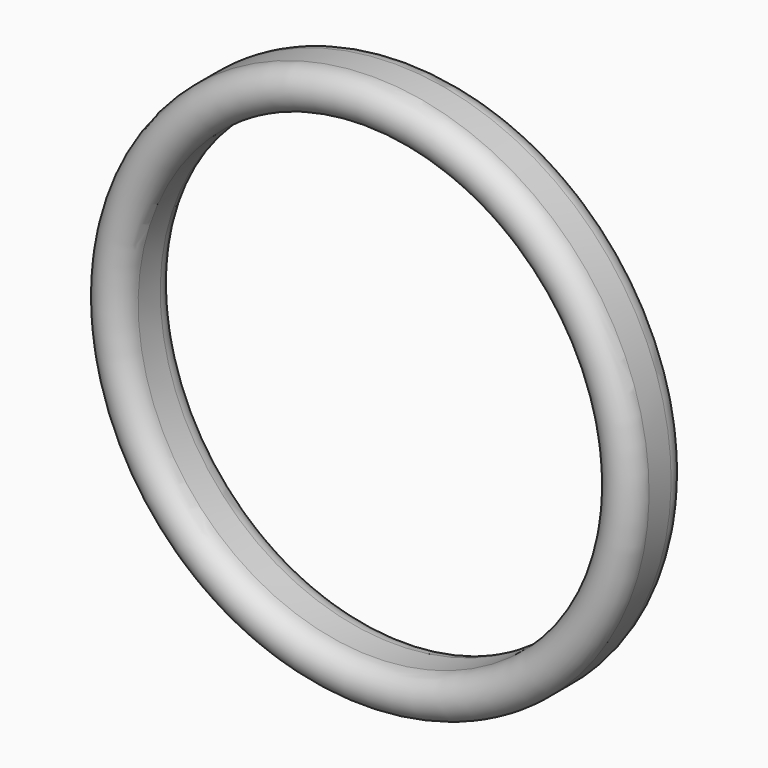
from build123d import *

# Parameters (mm, degrees)
F5_DEPTH = 6


# Not quite as in the source:
# - a feature of the source that left no trace in its solid (it failed there, or was rolled back) is left out


with BuildPart() as f1:
    # F0 (on Right) → F1 (revolve)
    with BuildSketch(Plane.YZ):
        with BuildLine():
            ThreePointArc((1.75, 29.85), (4.375, 32.475), (1.75, 35.1))
            Line((1.75, 35.1), (-1.75, 35.1))
            ThreePointArc((-1.75, 35.1), (-4.375, 32.475), (-1.75, 29.85))
            Line((-1.75, 29.85), (1.75, 29.85))
        make_face()
    revolve(axis=Axis((0, -4.6846177429, 0), (0, -1, 0)))


with BuildPart() as f3:
    # F2 (on Right) → F3 (revolve)
    with BuildSketch(Plane.YZ):
        with BuildLine():
            ThreePointArc((4.3570501582, 32.1685453172), (3.4944456795, 30.5134867395), (1.75, 29.85))
            Line((1.75, 29.85), (-1.75, 29.85))
            ThreePointArc((-1.75, 29.85), (-3.6061553006, 30.6188446994), (-4.375, 32.475))
            Line((-4.375, 32.475), (-4.375, 27.1685775369))
            Line((-4.375, 27.1685775369), (4.375, 27.1685775369))
            Line((4.375, 27.1685775369), (4.3570501582, 32.1685453172))
        make_face()
    revolve(axis=Axis((0, -6.0206142662, 0), (0, -1, 0)))

    # F4 (on Front) → F5 (join, symmetric)
    with BuildSketch(Plane.XZ):
        with BuildLine():
            ThreePointArc((-0.8, -1.805720078), (-1.9541006025, -0.286558607), (-1.2847665158, 1.5))
            Line((-1.2847665158, 1.5), (1.2847665158, 1.5))
            ThreePointArc((1.2847665158, 1.5), (1.9541006025, -0.286558607), (0.8, -1.805720078))
            Line((0.8, -1.805720078), (0.8, -6.9541354603))
            ThreePointArc((0.8, -6.9541354603), (2.1957679989, -6.6466986463), (3.5, -6.0621778265))
            ThreePointArc((3.5, -6.0621778265), (3.694735219, -5.9454967548), (3.8855844605, -5.8225624428))
            ThreePointArc((3.8855844605, -5.8225624428), (3.8880716888, -5.8324992461), (3.890563158, -5.8424349868))
            ThreePointArc((3.890563158, -5.8424349868), (8.500978981, -15.0837914383), (16.568096168, -21.5320643401))
            ThreePointArc((16.568096168, -21.5320643401), (18.1794560768, -20.1900713752), (19.6825117076, -18.727795873))
            ThreePointArc((19.6825117076, -18.727795873), (11.7812454852, -13.0384635672), (7.4660124048, -4.3105042717))
            ThreePointArc((7.4660124048, -4.3105042717), (17.1822634181, -3.6836260948), (26.0600028367, -7.6816572125))
            ThreePointArc((26.0600028367, -7.6816572125), (26.5748427535, -5.6488351019), (26.9313627985, -3.5823600038))
            ThreePointArc((26.9313627985, -3.5823600038), (17.3134360615, 0.1798319646), (7.0049786976, -0.4481090365))
            ThreePointArc((7.0049786976, -0.4481090365), (6.9951283591, -0.4509192312), (6.9852792208, -0.4537336299))
            ThreePointArc((6.9852792208, -0.4537336299), (6.9963188373, -0.2269861825), (7, 0))
            ThreePointArc((7, 0), (6.0621778265, 3.5), (3.5, 6.0621778265))
            ThreePointArc((3.5, 6.0621778265), (3.3015836183, 6.1724829373), (3.0996947604, 6.2762960727))
            ThreePointArc((3.0996947604, 6.2762960727), (3.1070566702, 6.2834184773), (3.1144155395, 6.2905440233))
            ThreePointArc((3.1144155395, 6.2905440233), (8.8124570805, 14.9039594738), (10.3632666305, 25.1144243439))
            ThreePointArc((10.3632666305, 25.1144243439), (8.3953866767, 25.838906477), (6.3774911291, 26.4094530856))
            ThreePointArc((6.3774911291, 26.4094530856), (5.4010179329, 16.722089662), (0, 8.6210085433))
            ThreePointArc((0, 8.6210085433), (-5.4010179329, 16.722089662), (-6.3774911291, 26.4094530856))
            ThreePointArc((-6.3774911291, 26.4094530856), (-8.3953866767, 25.838906477), (-10.3632666305, 25.1144243439))
            ThreePointArc((-10.3632666305, 25.1144243439), (-8.8124570805, 14.9039594738), (-3.1144155395, 6.2905440233))
            ThreePointArc((-3.1144155395, 6.2905440233), (-3.1070566702, 6.2834184773), (-3.0996947604, 6.2762960727))
            ThreePointArc((-3.0996947604, 6.2762960727), (-3.3015836183, 6.1724829373), (-3.5, 6.0621778265))
            ThreePointArc((-3.5, 6.0621778265), (-6.0621778265, 3.5), (-7, 0))
            ThreePointArc((-7, 0), (-6.9963188373, -0.2269861825), (-6.9852792208, -0.4537336299))
            ThreePointArc((-6.9852792208, -0.4537336299), (-6.9951283591, -0.4509192312), (-7.0049786976, -0.4481090365))
            ThreePointArc((-7.0049786976, -0.4481090365), (-17.3134360615, 0.1798319646), (-26.9313627985, -3.5823600038))
            ThreePointArc((-26.9313627985, -3.5823600038), (-26.5748427535, -5.6488351019), (-26.0600028367, -7.6816572125))
            ThreePointArc((-26.0600028367, -7.6816572125), (-17.1822634181, -3.6836260948), (-7.4660124048, -4.3105042717))
            ThreePointArc((-7.4660124048, -4.3105042717), (-11.7812454852, -13.0384635672), (-19.6825117076, -18.727795873))
            ThreePointArc((-19.6825117076, -18.727795873), (-18.1794560768, -20.1900713752), (-16.568096168, -21.5320643401))
            ThreePointArc((-16.568096168, -21.5320643401), (-8.500978981, -15.0837914383), (-3.890563158, -5.8424349868))
            ThreePointArc((-3.890563158, -5.8424349868), (-3.8880716888, -5.8324992461), (-3.8855844605, -5.8225624428))
            ThreePointArc((-3.8855844605, -5.8225624428), (-3.694735219, -5.9454967548), (-3.5, -6.0621778265))
            ThreePointArc((-3.5, -6.0621778265), (-2.1957679989, -6.6466986463), (-0.8, -6.9541354603))
            Line((-0.8, -6.9541354603), (-0.8, -1.805720078))
        make_face()
    extrude(amount=F5_DEPTH, both=True)

    # F6 (on Right) → F7 (revolve, cut)
    with BuildSketch(Plane.YZ):
        with BuildLine():
            Line((-13.0535820499, 2.701601783), (-6, 4))
            ThreePointArc((-6, 4), (-1.8810208663, 15.3523786055), (-4.375, 27.1685775369))
            Line((-4.375, 27.1685775369), (-11.726167053, 27.1685775369))
            Line((-11.726167053, 27.1685775369), (-13.0535820499, 2.701601783))
        make_face()
        with BuildLine():
            Line((12.8782450573, 27.7328483518), (4.375, 27.1685775369))
            ThreePointArc((4.375, 27.1685775369), (1.8810208663, 15.3523786055), (6, 4))
            Line((6, 4), (14.3638671536, 5.3453556511))
            Line((14.3638671536, 5.3453556511), (12.8782450573, 27.7328483518))
        make_face()
    revolve(axis=Axis((0, -4.9612242728, 0), (0, 1, 0)), mode=Mode.SUBTRACT)


solid = f1.part
